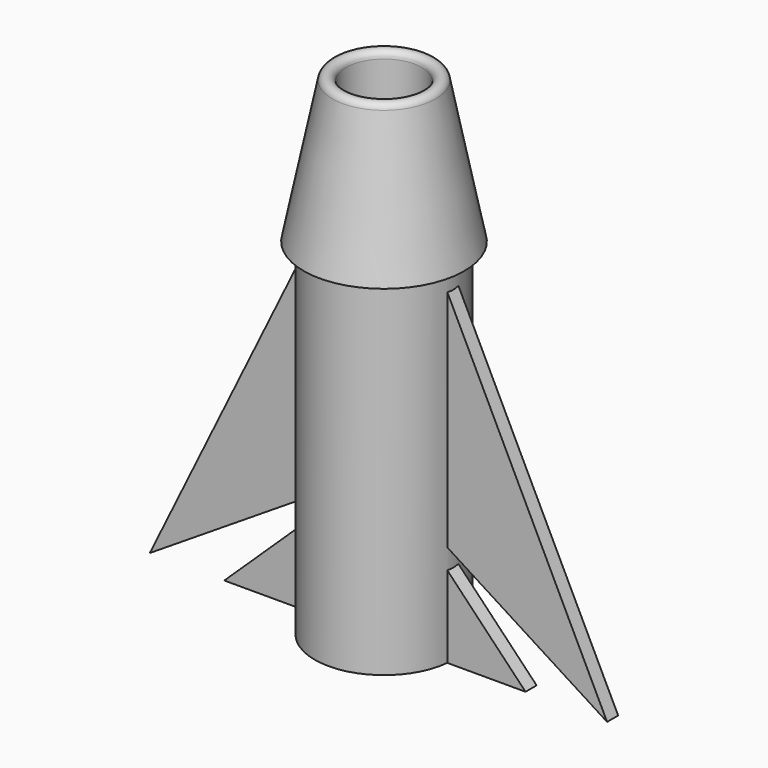
from build123d import *

# Parameters (mm, degrees)
F0_R        = 10
F1_DEPTH    = 50
F5_DEPTH    = 1
F7_R        = 5.4805132886
F8_DEPTH    = 107.4792907963
F9_T3_ANGLE = 270
F9_T6_ANGLE = 90


# Not quite as in the source:
# - a fillet or chamfer that OpenCascade refuses, or shapes differently, is made with other operations: its cross-section is extruded or revolved along the edge and cut away or added


with BuildPart() as f1:
    # F0 (on Top) → F1 (new body)
    with BuildSketch(Plane.XY):
        Circle(F0_R)
    extrude(amount=F1_DEPTH)

    # F4 (on Front) → F5 (join, symmetric)
    with BuildSketch(Plane.XZ):
        Polygon((-9.3656852841, 15.0750800967), (-9.0752122924, 48.9769205451), (-33.046875149, 0), align=None)
        Polygon((33.046875149, 0), (9.0752122924, 48.9769205451), (9.3656852841, 15.0750800967), align=None)
        Polygon((-9.8870191723, 11.8531188655), (-22.2848262638, 0), (-9.8870191723, 0), align=None)
        Polygon((21.2586894631, 0), (9.8870191723, 11.8531188655), (9.8870191723, 0), align=None)
    extrude(amount=F5_DEPTH, both=True)


with BuildPart() as f3:
    # F2 (on Right) → F3 (revolve)
    with BuildSketch(Plane.YZ):
        Polygon((0, 50), (11.6124056444, 50), (0, 107.4782907963), align=None)
    revolve(axis=Axis((0, 0, 78.7391453981), (0, 0, 1)))

    # F7 (on face) → F8 (cut, through all)
    with BuildSketch(Plane.XY.offset(107.4782907963)):
        Circle(F7_R)
    extrude(amount=-F8_DEPTH, mode=Mode.SUBTRACT)

    # F9: fillet of radius 1 on 2 edges, made by hand


with BuildPart() as f9_tool1:
    # F9_s2 → F9_t3 (revolve)
    with BuildSketch(Plane.YZ):
        with BuildLine():
            ThreePointArc((7.4607092239, 70.5497828324), (6.3810043326, 71.3467893791), (5.4805132886, 70.3517527126))
            Line((5.4805132886, 70.3517527126), (5.4805132886, 80.3512211639))
            Line((5.4805132886, 80.3512211639), (7.4607092239, 70.5497828324))
        make_face()
    revolve(axis=Axis((0, 0, 80.3512211639), (0, 0, 1)), revolution_arc=F9_T3_ANGLE)


with BuildPart() as f9_tool4:
    # F9_s5 → F9_t6 (revolve)
    with BuildSketch(Plane.XZ):
        with BuildLine():
            ThreePointArc((7.4607092239, 70.5497828324), (6.3810043326, 71.3467893791), (5.4805132886, 70.3517527126))
            Line((5.4805132886, 70.3517527126), (5.4805132886, 80.3512211639))
            Line((5.4805132886, 80.3512211639), (7.4607092239, 70.5497828324))
        make_face()
    revolve(axis=Axis((0, 0, 80.3512211639), (0, 0, 1)), revolution_arc=F9_T6_ANGLE)


with BuildPart() as f3_1:
    add(f3.part)

    # F9_t7: cut F9_tool1, F9_tool4
    add([f9_tool1.part, f9_tool4.part], mode=Mode.SUBTRACT)


solid = Compound([f1.part, f3_1.part])
